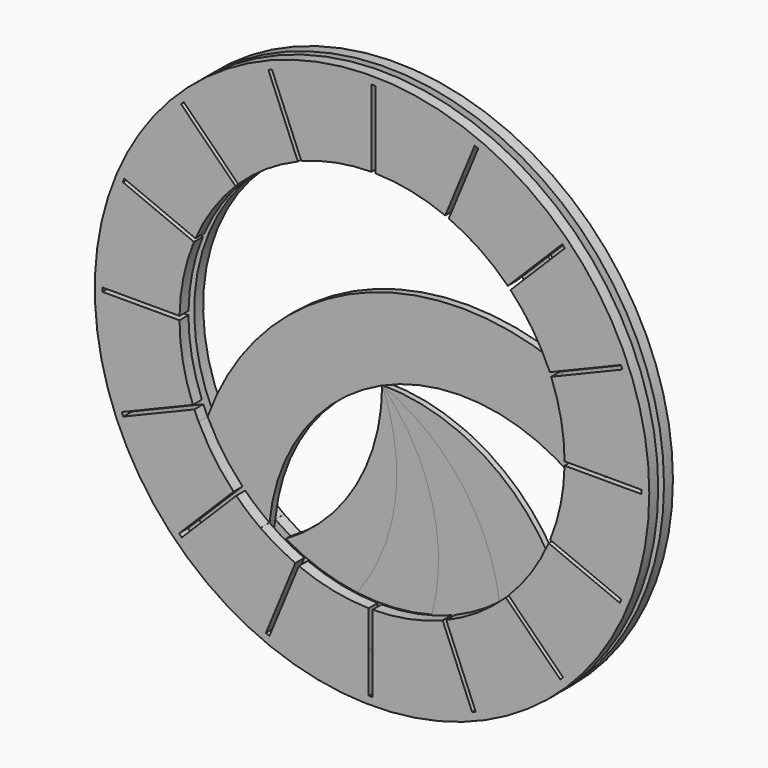
from build123d import *

# Parameters (mm, degrees)
F0_R      = 457.2
F0_R_2    = 444.5
F0_R_3    = 3.175
F1_DEPTH  = 18.415
F2_DEPTH  = 11.90625
F4_START  = 11.90625
F3_R      = 457.2
F3_R_2    = 3.175
F4_DEPTH  = 18.415
F5_R      = 3.175
F6_DEPTH  = 9.525
F7_DEPTH  = 9.525
F8_DEPTH  = 25.4
F9_DEPTH  = 9.525
F10_DEPTH = 9.525


with BuildPart() as f1:
    # F0 (on Front) → F1 (new body)
    with BuildSketch(Plane.XZ):
        Circle(F0_R)
        Circle(F0_R_2, mode=Mode.SUBTRACT)
        Circle(F0_R_2)
        with Locations((-145.8023877311, -351.9981018868)):
            Circle(F0_R_3, mode=Mode.SUBTRACT)
        with Locations((-351.9981018868, -145.8023877311)):
            Circle(F0_R_3, mode=Mode.SUBTRACT)
        with Locations((0, -381)):
            Circle(F0_R_3, mode=Mode.SUBTRACT)
        with Locations((145.8023877311, -351.9981018868)):
            Circle(F0_R_3, mode=Mode.SUBTRACT)
        with Locations((269.4076836321, -269.4076836321)):
            Circle(F0_R_3, mode=Mode.SUBTRACT)
        with BuildLine():
            ThreePointArc((422.4513888889, 48.1043902277), (438.7252682733, 26.4583333333), (444.5, 0))
            ThreePointArc((444.5, 0), (407.4583333333, -57.7252682733), (339.5486111111, -48.1043902277))
            ThreePointArc((339.5486111111, -48.1043902277), (328.041448396, -38.6497965609), (316.103577158, -29.7452266409))
            ThreePointArc((316.103577158, -29.7452266409), (132.2916666667, -288.6263413664), (-183.8119104913, -258.8811147255))
            ThreePointArc((-183.8119104913, -258.8811147255), (-183.9228426359, -260.0845455834), (-184.0291932426, -261.2883899749))
            ThreePointArc((-184.0291932426, -261.2883899749), (-252.7609555027, -319.0849716785), (-310.5575372063, -250.3532094184))
            ThreePointArc((-310.5575372063, -250.3532094184), (-301.8872628806, -193.3955315556), (-285.9227769911, -138.0377325143))
            ThreePointArc((-285.9227769911, -138.0377325143), (-132.2916666667, 288.6263413664), (291.2144436578, 126.4926788597))
            ThreePointArc((291.2144436578, 126.4926788596), (360.2279597917, 92.9824848895), (422.4513888889, 48.1043902277))
        make_face(mode=Mode.SUBTRACT)
        with Locations((351.9981018868, -145.8023877311)):
            Circle(F0_R_3, mode=Mode.SUBTRACT)
        with Locations((-381, 0)):
            Circle(F0_R_3, mode=Mode.SUBTRACT)
        with Locations((-351.9981018868, 145.8023877311)):
            Circle(F0_R_3, mode=Mode.SUBTRACT)
        with Locations((-269.4076836321, 269.4076836321)):
            Circle(F0_R_3, mode=Mode.SUBTRACT)
        with Locations((-145.8023877311, 351.9981018868)):
            Circle(F0_R_3, mode=Mode.SUBTRACT)
        with Locations((351.9981018868, 145.8023877311)):
            Circle(F0_R_3, mode=Mode.SUBTRACT)
        with Locations((0, 381)):
            Circle(F0_R_3, mode=Mode.SUBTRACT)
        with Locations((145.8023877311, 351.9981018868)):
            Circle(F0_R_3, mode=Mode.SUBTRACT)
        with Locations((269.4076836321, 269.4076836321)):
            Circle(F0_R_3, mode=Mode.SUBTRACT)
        with BuildLine():
            ThreePointArc((339.5486111111, -48.1043902277), (407.4583333333, -57.7252682733), (444.5, 0))
            ThreePointArc((444.5, 0), (438.7252682733, 26.4583333333), (422.4513888889, 48.1043902277))
            ThreePointArc((422.4513888889, 48.1043902277), (360.2279597917, 92.9824848895), (291.2144436578, 126.4926788596))
            ThreePointArc((291.2144436578, 126.4926788597), (310.8591609245, 64.597461787), (317.5, 0))
            ThreePointArc((317.5, 0), (317.1507021494, -14.8889934572), (316.103577158, -29.7452266409))
            ThreePointArc((316.103577158, -29.7452266409), (328.041448396, -38.6497965609), (339.5486111111, -48.1043902277))
        make_face()
        with Locations((381, 0)):
            Circle(F0_R_3, mode=Mode.SUBTRACT)
        with BuildLine():
            ThreePointArc((-183.8653331924, -258.8431750115), (-242.5359887763, -204.8964229759), (-285.9227769911, -138.0377325143))
            ThreePointArc((-285.9227769911, -138.0377325143), (-301.8872628806, -193.3955315556), (-310.5575372063, -250.3532094184))
            ThreePointArc((-310.5575372063, -250.3532094184), (-252.7609555027, -319.0849716785), (-184.0291932426, -261.2883899749))
            ThreePointArc((-184.0291932426, -261.2883899749), (-183.9354658864, -260.0665730623), (-183.8653331924, -258.8431750115))
        make_face()
        with Locations((-269.4076836321, -269.4076836321)):
            Circle(F0_R_3, mode=Mode.SUBTRACT)
        with Locations((-247.2933652244, -255.8207996967)):
            Circle(F0_R_3, mode=Mode.SUBTRACT)
        with Locations((-247.2933652244, -255.8207996967)):
            Circle(F0_R_3)
    extrude(amount=-F1_DEPTH)


with BuildPart() as f2:
    # F0 (on Front) → F2 (new body)
    with BuildSketch(Plane.XZ):
        with BuildLine():
            ThreePointArc((-183.8119104913, -258.8811147255), (0, 0), (316.103577158, -29.7452266409))
            ThreePointArc((316.103577158, -29.7452266409), (317.1507021494, -14.8889934572), (317.5, 0))
            ThreePointArc((317.5, 0), (310.8591609245, 64.597461787), (291.2144436578, 126.4926788597))
            ThreePointArc((291.2144436578, 126.4926788596), (-52.9166666667, 115.4505365466), (-285.9227769911, -138.0377325143))
            ThreePointArc((-285.9227769911, -138.0377325143), (-242.5359887763, -204.8964229759), (-183.8653331924, -258.8431750115))
            ThreePointArc((-183.8653331924, -258.8431750115), (-183.8386228206, -258.8621462467), (-183.8119104913, -258.8811147255))
        make_face()
        with BuildLine():
            ThreePointArc((339.5486111111, -48.1043902277), (407.4583333333, -57.7252682733), (444.5, 0))
            ThreePointArc((444.5, 0), (438.7252682733, 26.4583333333), (422.4513888889, 48.1043902277))
            ThreePointArc((422.4513888889, 48.1043902277), (360.2279597917, 92.9824848895), (291.2144436578, 126.4926788596))
            ThreePointArc((291.2144436578, 126.4926788597), (310.8591609245, 64.597461787), (317.5, 0))
            ThreePointArc((317.5, 0), (317.1507021494, -14.8889934572), (316.103577158, -29.7452266409))
            ThreePointArc((316.103577158, -29.7452266409), (328.041448396, -38.6497965609), (339.5486111111, -48.1043902277))
        make_face()
        with Locations((381, 0)):
            Circle(F0_R_3, mode=Mode.SUBTRACT)
        with BuildLine():
            ThreePointArc((-183.8653331924, -258.8431750115), (-242.5359887763, -204.8964229759), (-285.9227769911, -138.0377325143))
            ThreePointArc((-285.9227769911, -138.0377325143), (-301.8872628806, -193.3955315556), (-310.5575372063, -250.3532094184))
            ThreePointArc((-310.5575372063, -250.3532094184), (-252.7609555027, -319.0849716785), (-184.0291932426, -261.2883899749))
            ThreePointArc((-184.0291932426, -261.2883899749), (-183.9354658864, -260.0665730623), (-183.8653331924, -258.8431750115))
        make_face()
        with Locations((-269.4076836321, -269.4076836321)):
            Circle(F0_R_3, mode=Mode.SUBTRACT)
        with Locations((-247.2933652244, -255.8207996967)):
            Circle(F0_R_3, mode=Mode.SUBTRACT)
        with Locations((-269.4076836321, -269.4076836321)):
            Circle(F0_R_3)
    extrude(amount=F2_DEPTH)


with BuildPart() as f4:
    # F3 (on Front) → F4 (new body)
    with BuildSketch(Plane.XZ.offset(F4_START)):
        Circle(F3_R)
        with BuildLine():
            ThreePointArc((444.4991019176, 0.893529228), (444.4997754793, 0.4467648397), (444.5, 0))
            ThreePointArc((444.5, 0), (444.4916269754, -2.7282867786), (444.4665082171, -5.456470772))
            ThreePointArc((444.4665082171, -5.456470772), (435.5082100725, -88.9541958505), (411.0055613132, -169.2769286396))
            ThreePointArc((411.0055613132, -169.2769286396), (409.7859392208, -172.208402864), (408.5454088649, -175.1310906019))
            ThreePointArc((408.5454088649, -175.1310906019), (368.3158245353, -248.844737531), (314.9401497735, -313.6765086209))
            ThreePointArc((314.9401497735, -313.6765086209), (312.6915392669, -315.9181084884), (310.4269744864, -318.1435894549))
            ThreePointArc((310.4269744864, -318.1435894549), (245.0506935038, -370.8509237056), (170.9279553705, -410.3216836494))
            ThreePointArc((170.9279553705, -410.3216836494), (167.9926870155, -411.5321459003), (165.0488472698, -412.7216107922))
            ThreePointArc((165.0488472698, -412.7216107922), (84.4788157765, -436.398418518), (0.893529228, -444.4991019176))
            ThreePointArc((0.893529228, -444.4991019176), (-2.2815289766, -444.4941446471), (-5.456470772, -444.4665082171))
            ThreePointArc((-5.456470772, -444.4665082171), (-88.9541958505, -435.5082100725), (-169.2769286396, -411.0055613132))
            ThreePointArc((-169.2769286396, -411.0055613132), (-172.208402864, -409.7859392208), (-175.1310906019, -408.5454088649))
            ThreePointArc((-175.1310906019, -408.5454088649), (-248.844737531, -368.3158245353), (-313.6765086209, -314.9401497735))
            ThreePointArc((-313.6765086209, -314.9401497735), (-315.9181084884, -312.6915392669), (-318.1435894549, -310.4269744864))
            ThreePointArc((-318.1435894549, -310.4269744864), (-370.8509237056, -245.0506935038), (-410.3216836494, -170.9279553705))
            ThreePointArc((-410.3216836494, -170.9279553705), (-411.5321459003, -167.9926870155), (-412.7216107922, -165.0488472698))
            ThreePointArc((-412.7216107922, -165.0488472698), (-436.398418518, -84.4788157765), (-444.4991019176, -0.893529228))
            ThreePointArc((-444.4991019176, -0.893529228), (-444.4941446471, 2.2815289766), (-444.4665082171, 5.456470772))
            ThreePointArc((-444.4665082171, 5.456470772), (-435.5082100725, 88.9541958505), (-411.0055613132, 169.2769286396))
            ThreePointArc((-411.0055613132, 169.2769286396), (-409.7859392208, 172.208402864), (-408.5454088649, 175.1310906019))
            ThreePointArc((-408.5454088649, 175.1310906019), (-368.3158245353, 248.844737531), (-314.9401497735, 313.6765086209))
            ThreePointArc((-314.9401497735, 313.6765086209), (-312.6915392669, 315.9181084884), (-310.4269744864, 318.1435894549))
            ThreePointArc((-310.4269744864, 318.1435894549), (-245.0506935038, 370.8509237056), (-170.9279553705, 410.3216836494))
            ThreePointArc((-170.9279553705, 410.3216836494), (-167.9926870155, 411.5321459003), (-165.0488472698, 412.7216107922))
            ThreePointArc((-165.0488472698, 412.7216107922), (-84.4788157765, 436.398418518), (-0.893529228, 444.4991019176))
            ThreePointArc((-0.893529228, 444.4991019176), (2.2815289766, 444.4941446471), (5.456470772, 444.4665082171))
            ThreePointArc((5.456470772, 444.4665082171), (88.9541958505, 435.5082100725), (169.2769286396, 411.0055613132))
            ThreePointArc((169.2769286396, 411.0055613132), (172.208402864, 409.7859392208), (175.1310906019, 408.5454088649))
            ThreePointArc((175.1310906019, 408.5454088649), (248.844737531, 368.3158245353), (313.6765086209, 314.9401497735))
            ThreePointArc((313.6765086209, 314.9401497735), (315.9181084884, 312.6915392669), (318.1435894549, 310.4269744864))
            ThreePointArc((318.1435894549, 310.4269744864), (370.8509237056, 245.0506935038), (410.3216836494, 170.9279553705))
            ThreePointArc((410.3216836494, 170.9279553705), (411.5321459003, 167.9926870155), (412.7216107922, 165.0488472698))
            ThreePointArc((412.7216107922, 165.0488472698), (436.398418518, 84.4788157765), (444.4991019176, 0.893529228))
        make_face(mode=Mode.SUBTRACT)
        with BuildLine():
            ThreePointArc((0.893529228, -444.4991019176), (84.4788157765, -436.398418518), (165.0488472698, -412.7216107922))
            Line((165.0488472698, -412.7216107922), (116.4429240103, -295.3765316472))
            ThreePointArc((116.4429240103, -295.3765316472), (59.7018330532, -311.8364012268), (0.893529228, -317.4987426834))
            Line((0.893529228, -317.4987426834), (0.893529228, -444.4991019176))
        make_face()
        with BuildLine():
            ThreePointArc((-5.456470772, -317.4531098079), (-64.1773227466, -310.9461709767), (-120.6759952562, -293.6725287951))
            Line((-120.6759952562, -293.6725287951), (-169.2769286396, -411.0055613132))
            ThreePointArc((-169.2769286396, -411.0055613132), (-88.9541958505, -435.5082100725), (-5.456470772, -444.4665082171))
            Line((-5.456470772, -444.4665082171), (-5.456470772, -379.1493962176))
            ThreePointArc((-5.456470772, -379.1493962176), (-5.4858422756, -378.718529228), (-5.456470772, -378.2876622384))
            Line((-5.456470772, -378.2876622384), (-5.456470772, -317.4531098079))
        make_face()
        with BuildLine():
            ThreePointArc((170.9279553705, -410.3216836494), (245.0506935038, -370.8509237056), (310.4269744864, -318.1435894549))
            Line((310.4269744864, -318.1435894549), (220.6149391697, -228.3315541382))
            ThreePointArc((220.6149391697, -228.3315541382), (174.4919259691, -265.2523661941), (122.3270219871, -292.9886511313))
            Line((122.3270219871, -292.9886511313), (144.9919439166, -347.7066130437))
            ThreePointArc((144.9919439166, -347.7066130437), (146.3432423245, -348.8781658945), (146.8469499574, -350.5942142883))
            ThreePointArc((146.8469499574, -350.5942142883), (146.7966055901, -351.1573769442), (146.6471690585, -351.70268003))
            Line((146.6471690585, -351.70268003), (170.9279553705, -410.3216836494))
        make_face()
        with BuildLine():
            Line((146.6307933887, 356.3329544552), (169.2769286396, 411.0055613132))
            ThreePointArc((169.2769286396, 411.0055613132), (88.9541958505, 435.5082100725), (5.456470772, 444.4665082171))
            Line((5.456470772, 444.4665082171), (5.456470772, 383.3108422756))
            Line((5.456470772, 383.3108422756), (5.456470772, 317.4531098079))
            ThreePointArc((5.456470772, 317.4531098079), (64.1773227466, 310.9461709767), (120.6759952562, 293.6725287951))
            Line((120.6759952562, 293.6725287951), (144.9535218219, 352.2836626909))
            ThreePointArc((144.9535218219, 352.2836626909), (144.9813764733, 354.6441451141), (146.6307933887, 356.3329544552))
        make_face()
        with BuildLine():
            Line((-0.893529228, 383.3108422756), (-0.893529228, 444.4991019176))
            ThreePointArc((-0.893529228, 444.4991019176), (-84.4788157765, 436.398418518), (-165.0488472698, 412.7216107922))
            Line((-165.0488472698, 412.7216107922), (-142.4203824907, 358.0916642267))
            ThreePointArc((-142.4203824907, 358.0916642267), (-141.0416592427, 356.9205463337), (-140.526321461, 355.1865273359))
            ThreePointArc((-140.526321461, 355.1865273359), (-140.5805336323, 354.6023113415), (-140.7413188331, 354.0380459723))
            Line((-140.7413188331, 354.0380459723), (-116.4429240103, 295.3765316472))
            ThreePointArc((-116.4429240103, 295.3765316472), (-59.7018330532, 311.8364012268), (-0.893529228, 317.4987426834))
            Line((-0.893529228, 317.4987426834), (-0.893529228, 383.3108422756))
        make_face()
        with BuildLine():
            ThreePointArc((314.9401497735, -313.6765086209), (368.3158245353, -248.844737531), (408.5454088649, -175.1310906019))
            Line((408.5454088649, -175.1310906019), (291.20032972, -126.5251673423))
            ThreePointArc((291.20032972, -126.5251673423), (262.7172049295, -178.2860629271), (225.1373345459, -223.8736933933))
            Line((225.1373345459, -223.8736933933), (266.9456916083, -265.6820504557))
            ThreePointArc((266.9456916083, -265.6820504557), (269.7075090207, -266.2227656353), (270.9547544263, -268.7455393516))
            ThreePointArc((270.9547544263, -268.7455393516), (270.9267531747, -269.1662814076), (270.8432433222, -269.5796021696))
            Line((270.8432433222, -269.5796021696), (314.9401497735, -313.6765086209))
        make_face()
        with BuildLine():
            Line((271.8840859169, 273.1477270695), (313.6765086209, 314.9401497735))
            ThreePointArc((313.6765086209, 314.9401497735), (248.844737531, 368.3158245353), (175.1310906019, 408.5454088649))
            Line((175.1310906019, 408.5454088649), (126.5251673423, 291.20032972))
            ThreePointArc((126.5251673423, 291.20032972), (178.2860629271, 262.7172049295), (223.8736933933, 225.1373345459))
            Line((223.8736933933, 225.1373345459), (267.969879756, 269.2335209086))
            ThreePointArc((267.969879756, 269.2335209086), (268.7819460933, 272.3356607322), (271.8840859169, 273.1477270695))
        make_face()
        with BuildLine():
            Line((-122.3270219871, 292.9886511313), (-170.9279553705, 410.3216836494))
            ThreePointArc((-170.9279553705, 410.3216836494), (-245.0506935038, 370.8509237056), (-310.4269744864, 318.1435894549))
            Line((-310.4269744864, 318.1435894549), (-268.6756914301, 276.3923063985))
            ThreePointArc((-268.6756914301, 276.3923063985), (-265.8948010441, 275.8708319158), (-264.6341259299, 273.3378523992))
            ThreePointArc((-264.6341259299, 273.3378523992), (-264.664406829, 272.9003975146), (-264.7546719306, 272.4712868991))
            Line((-264.7546719306, 272.4712868991), (-220.6149391697, 228.3315541382))
            ThreePointArc((-220.6149391697, 228.3315541382), (-174.4919259691, 265.2523661941), (-122.3270219871, 292.9886511313))
        make_face()
        with BuildLine():
            Line((-347.9778941764, 150.0432045786), (-291.20032972, 126.5251673423))
            ThreePointArc((-291.20032972, 126.5251673423), (-262.7172049295, 178.2860629271), (-225.1373345459, 223.8736933933))
            Line((-225.1373345459, 223.8736933933), (-314.9401497735, 313.6765086209))
            ThreePointArc((-314.9401497735, 313.6765086209), (-368.3158245353, 248.844737531), (-408.5454088649, 175.1310906019))
            Line((-408.5454088649, 175.1310906019), (-353.5179413961, 152.3379672732))
            ThreePointArc((-353.5179413961, 152.3379672732), (-350.0173969675, 153.1925453708), (-347.9726544443, 150.2255362646))
            ThreePointArc((-347.9726544443, 150.2255362646), (-347.9739646477, 150.1343327854), (-347.9778941764, 150.0432045786))
        make_face()
        with BuildLine():
            Line((-350.5268722304, -139.2869430493), (-295.3765316472, -116.4429240103))
            ThreePointArc((-295.3765316472, -116.4429240103), (-311.8364012268, -59.7018330532), (-317.4987426834, -0.893529228))
            Line((-317.4987426834, -0.893529228), (-444.4991019176, -0.893529228))
            ThreePointArc((-444.4991019176, -0.893529228), (-436.398418518, -84.4788157765), (-412.7216107922, -165.0488472698))
            Line((-412.7216107922, -165.0488472698), (-356.0741114993, -141.5846847882))
            ThreePointArc((-356.0741114993, -141.5846847882), (-354.1200764617, -138.4571616697), (-350.5268722304, -139.2869430493))
        make_face()
        with BuildLine():
            Line((-377.9742354301, 5.456470772), (-317.4531098079, 5.456470772))
            ThreePointArc((-317.4531098079, 5.456470772), (-310.9461709767, 64.1773227466), (-293.6725287951, 120.6759952562))
            Line((-293.6725287951, 120.6759952562), (-411.0055613132, 169.2769286396))
            ThreePointArc((-411.0055613132, 169.2769286396), (-435.5082100725, 88.9541958505), (-444.4665082171, 5.456470772))
            Line((-444.4665082171, 5.456470772), (-384.0845075771, 5.456470772))
            ThreePointArc((-384.0845075771, 5.456470772), (-381.0293715036, 7.7673130476), (-377.9742354301, 5.456470772))
        make_face()
        with BuildLine():
            Line((355.2331404575, 148.109533649), (410.3216836494, 170.9279553705))
            ThreePointArc((410.3216836494, 170.9279553705), (370.8509237056, 245.0506935038), (318.1435894549, 310.4269744864))
            Line((318.1435894549, 310.4269744864), (228.3315541382, 220.6149391697))
            ThreePointArc((228.3315541382, 220.6149391697), (264.0014411474, 176.3788226293), (291.2144436578, 126.4926788596))
            ThreePointArc((291.2144436578, 126.4926788596), (294.2607523904, 125.3135881763), (297.2983140397, 124.112142813))
            Line((297.2983140397, 124.112142813), (349.7048790855, 145.8196528124))
            ThreePointArc((349.7048790855, 145.8196528124), (351.6606651625, 148.9161097488), (355.2331404575, 148.109533649))
        make_face()
        with BuildLine():
            ThreePointArc((411.0055613132, -169.2769286396), (435.5082100725, -88.9541958505), (444.4665082171, -5.456470772))
            Line((444.4665082171, -5.456470772), (444.2651319979, -5.456470772))
            ThreePointArc((444.2651319979, -5.456470772), (404.951432224, -58.8096836789), (339.5486111111, -48.1043902277))
            ThreePointArc((339.5486111111, -48.1043902277), (328.041448396, -38.6497965609), (316.103577158, -29.7452266409))
            ThreePointArc((316.103577158, -29.7452266409), (308.2593486305, -76.0422512944), (293.6725287951, -120.6759952562))
            Line((293.6725287951, -120.6759952562), (348.7688393659, -143.4976343313))
            ThreePointArc((348.7688393659, -143.4976343313), (352.2630845938, -142.6717954912), (354.2932829407, -145.633223217))
            ThreePointArc((354.2932829407, -145.633223217), (354.2923820296, -145.7088537277), (354.2896798074, -145.7844413179))
            Line((354.2896798074, -145.7844413179), (411.0055613132, -169.2769286396))
        make_face()
        with BuildLine():
            ThreePointArc((-126.5251673423, -291.20032972), (-156.0077189886, -276.5281931666), (-183.8119104913, -258.8811147255))
            ThreePointArc((-183.8119104913, -258.8811147255), (-183.9228426359, -260.0845455834), (-184.0291932426, -261.2883899749))
            ThreePointArc((-184.0291932426, -261.2883899749), (-227.9761851143, -316.3112663224), (-295.6794161791, -296.9430573317))
            Line((-295.6794161791, -296.9430573317), (-313.6765086209, -314.9401497735))
            ThreePointArc((-313.6765086209, -314.9401497735), (-248.844737531, -368.3158245353), (-175.1310906019, -408.5454088649))
            Line((-175.1310906019, -408.5454088649), (-150.889729434, -350.0215859632))
            ThreePointArc((-150.889729434, -350.0215859632), (-150.8773830083, -347.621792271), (-149.1892028564, -345.9161516364))
            Line((-149.1892028564, -345.9161516364), (-126.5251673423, -291.20032972))
        make_face()
        with BuildLine():
            ThreePointArc((-310.5575372063, -250.3532094184), (-301.8872628806, -193.3955315555), (-285.9227769911, -138.0377325143))
            ThreePointArc((-285.9227769911, -138.0377325143), (-289.5622851979, -130.2303074978), (-292.9886511313, -122.3270219871))
            Line((-292.9886511313, -122.3270219871), (-410.3216836494, -170.9279553705))
            ThreePointArc((-410.3216836494, -170.9279553705), (-370.8509237056, -245.0506935038), (-318.1435894549, -310.4269744864))
            Line((-318.1435894549, -310.4269744864), (-299.5759800047, -291.8593650362))
            ThreePointArc((-299.5759800047, -291.8593650362), (-308.6811101032, -272.062560029), (-310.5575372063, -250.3532094184))
        make_face()
        with BuildLine():
            Line((384.0466753222, 0.893529228), (444.4937131181, 0.893529228))
            ThreePointArc((444.4937131181, 0.893529228), (438.5376829382, 26.863824041), (422.4513888889, 48.1043902277))
            ThreePointArc((422.4513888889, 48.1043902277), (366.8608063144, 88.9416243363), (305.6214900159, 120.6865247125))
            Line((305.6214900159, 120.6865247125), (295.3765316472, 116.4429240103))
            ThreePointArc((295.3765316472, 116.4429240103), (311.8364012268, 59.7018330532), (317.4987426834, 0.893529228))
            Line((317.4987426834, 0.893529228), (377.9533246778, 0.893529228))
            ThreePointArc((377.9533246778, 0.893529228), (381, 3.175), (384.0466753222, 0.893529228))
        make_face()
        with BuildLine():
            Line((444.4937131181, 0.893529228), (444.4991019176, 0.893529228))
            ThreePointArc((444.4991019176, 0.893529228), (436.398418518, 84.4788157765), (412.7216107922, 165.0488472698))
            Line((412.7216107922, 165.0488472698), (305.6214900159, 120.6865247125))
            ThreePointArc((305.6214900159, 120.6865247125), (366.8608063144, 88.9416243363), (422.4513888889, 48.1043902277))
            ThreePointArc((422.4513888889, 48.1043902277), (438.5376829382, 26.863824041), (444.4937131181, 0.893529228))
        make_face()
        with BuildLine():
            ThreePointArc((-228.3315541382, -220.6149391697), (-260.4210591255, -181.6235721594), (-285.9227769911, -138.0377325143))
            ThreePointArc((-285.9227769911, -138.0377325143), (-301.8872628806, -193.3955315555), (-310.5575372063, -250.3532094184))
            ThreePointArc((-310.5575372063, -250.3532094184), (-308.6811101032, -272.062560029), (-299.5759800047, -291.8593650362))
            Line((-299.5759800047, -291.8593650362), (-274.1042725424, -266.387657574))
            ThreePointArc((-274.1042725424, -266.387657574), (-273.3014456575, -263.253219624), (-270.1670077076, -262.4503927391))
            Line((-270.1670077076, -262.4503927391), (-228.3315541382, -220.6149391697))
        make_face()
        with BuildLine():
            ThreePointArc((-184.0291932426, -261.2883899749), (-183.9354658864, -260.0665730623), (-183.8653331924, -258.8431750115))
            ThreePointArc((-183.8653331924, -258.8431750115), (-204.5649025875, -242.8156721247), (-223.8736933933, -225.1373345459))
            Line((-223.8736933933, -225.1373345459), (-295.6794161791, -296.9430573317))
            ThreePointArc((-295.6794161791, -296.9430573317), (-227.9761851143, -316.3112663224), (-184.0291932426, -261.2883899749))
        make_face()
        with Locations((-247.2933652244, -255.8207996967)):
            Circle(F3_R_2, mode=Mode.SUBTRACT)
        with BuildLine():
            ThreePointArc((339.5486111111, -48.1043902277), (404.951432224, -58.8096836789), (444.2651319979, -5.456470772))
            Line((444.2651319979, -5.456470772), (317.4531098079, -5.456470772))
            ThreePointArc((317.4531098079, -5.456470772), (317.0110484119, -17.6137782653), (316.103577158, -29.7452266409))
            ThreePointArc((316.103577158, -29.7452266409), (328.041448396, -38.6497965609), (339.5486111111, -48.1043902277))
        make_face()
        with Locations((-247.2933652244, -255.8207996967)):
            Circle(F3_R_2)
        with BuildLine():
            Line((292.9886511313, 122.3270219871), (297.2983140397, 124.112142813))
            ThreePointArc((297.2983140397, 124.112142813), (294.2607523904, 125.3135881763), (291.2144436578, 126.4926788596))
            ThreePointArc((291.2144436578, 126.4926788596), (292.1089730984, 124.4130131273), (292.9886511313, 122.3270219871))
        make_face()
        with BuildLine():
            Line((-384.0845075771, 5.456470772), (-377.9742354301, 5.456470772))
            ThreePointArc((-377.9742354301, 5.456470772), (-381.0293715036, 7.7673130476), (-384.0845075771, 5.456470772))
        make_face()
        with BuildLine():
            Line((377.9533246778, 0.893529228), (384.0466753222, 0.893529228))
            ThreePointArc((384.0466753222, 0.893529228), (381, 3.175), (377.9533246778, 0.893529228))
        make_face()
        with BuildLine():
            Line((-356.0741114993, -141.5846847882), (-350.5268722304, -139.2869430493))
            ThreePointArc((-350.5268722304, -139.2869430493), (-354.1200764617, -138.4571616697), (-356.0741114993, -141.5846847882))
        make_face()
        with BuildLine():
            Line((-353.5179413961, 152.3379672732), (-347.9778941764, 150.0432045786))
            ThreePointArc((-347.9778941764, 150.0432045786), (-347.9739646477, 150.1343327854), (-347.9726544443, 150.2255362646))
            ThreePointArc((-347.9726544443, 150.2255362646), (-350.0173969675, 153.1925453708), (-353.5179413961, 152.3379672732))
        make_face()
        with BuildLine():
            Line((349.7048790855, 145.8196528124), (355.2331404575, 148.109533649))
            ThreePointArc((355.2331404575, 148.109533649), (351.6606651625, 148.9161097488), (349.7048790855, 145.8196528124))
        make_face()
        with BuildLine():
            Line((348.7688393659, -143.4976343313), (354.2896798074, -145.7844413179))
            ThreePointArc((354.2896798074, -145.7844413179), (354.2923820296, -145.7088537277), (354.2932829407, -145.633223217))
            ThreePointArc((354.2932829407, -145.633223217), (352.2630845938, -142.6717954912), (348.7688393659, -143.4976343313))
        make_face()
        with BuildLine():
            Line((-274.1042725424, -266.387657574), (-270.1670077076, -262.4503927391))
            ThreePointArc((-270.1670077076, -262.4503927391), (-273.3014456575, -263.253219624), (-274.1042725424, -266.387657574))
        make_face()
        with BuildLine():
            ThreePointArc((-264.6341259299, 273.3378523992), (-265.8948010441, 275.8708319158), (-268.6756914301, 276.3923063985))
            Line((-268.6756914301, 276.3923063985), (-264.7546719306, 272.4712868991))
            ThreePointArc((-264.7546719306, 272.4712868991), (-264.664406829, 272.9003975146), (-264.6341259299, 273.3378523992))
        make_face()
        with BuildLine():
            Line((267.969879756, 269.2335209086), (271.8840859169, 273.1477270695))
            ThreePointArc((271.8840859169, 273.1477270695), (268.7819460933, 272.3356607322), (267.969879756, 269.2335209086))
        make_face()
        with BuildLine():
            Line((266.9456916083, -265.6820504557), (270.8432433222, -269.5796021696))
            ThreePointArc((270.8432433222, -269.5796021696), (270.9267531747, -269.1662814076), (270.9547544263, -268.7455393516))
            ThreePointArc((270.9547544263, -268.7455393516), (269.7075090207, -266.2227656353), (266.9456916083, -265.6820504557))
        make_face()
        with BuildLine():
            Line((-150.889729434, -350.0215859632), (-149.1892028564, -345.9161516364))
            ThreePointArc((-149.1892028564, -345.9161516364), (-150.8773830083, -347.621792271), (-150.889729434, -350.0215859632))
        make_face()
        with BuildLine():
            ThreePointArc((-140.526321461, 355.1865273359), (-141.0416592427, 356.9205463337), (-142.4203824907, 358.0916642267))
            Line((-142.4203824907, 358.0916642267), (-140.7413188331, 354.0380459723))
            ThreePointArc((-140.7413188331, 354.0380459723), (-140.5805336323, 354.6023113415), (-140.526321461, 355.1865273359))
        make_face()
        with BuildLine():
            Line((144.9535218219, 352.2836626909), (146.6307933887, 356.3329544552))
            ThreePointArc((146.6307933887, 356.3329544552), (144.9813764733, 354.6441451141), (144.9535218219, 352.2836626909))
        make_face()
        with BuildLine():
            Line((144.9919439166, -347.7066130437), (146.6471690585, -351.70268003))
            ThreePointArc((146.6471690585, -351.70268003), (146.7966055901, -351.1573769442), (146.8469499574, -350.5942142883))
            ThreePointArc((146.8469499574, -350.5942142883), (146.3432423245, -348.8781658945), (144.9919439166, -347.7066130437))
        make_face()
    extrude(amount=F4_DEPTH)


with BuildPart() as f6:
    # F5 (on Front) → F6 (new body)
    with BuildSketch(Plane.XZ):
        with BuildLine():
            ThreePointArc((71.7370250666, -375.0863708473), (104.2081806235, -413.9328112946), (154.7634294478, -416.6875698957))
            ThreePointArc((154.7634294478, -416.6875698957), (166.2544105163, -411.0429346054), (176.3796033569, -403.2080751032))
            ThreePointArc((176.3796033569, -403.2080751032), (186.4354217322, -370.6673875603), (192.9476872854, -337.2367694635))
            ThreePointArc((192.9476872854, -337.2367694635), (162.4728125061, -301.0973226443), (115.4717831233, -296.0296953712))
            ThreePointArc((115.4717831233, -296.0296953712), (95.6182169929, -336.6720898203), (71.7370250666, -375.0863708473))
        make_face()
        with Locations((132.6543703377, -357.1607733645)):
            Circle(F5_R, mode=Mode.SUBTRACT)
        with Locations((145.8023877311, -351.9981018868)):
            Circle(F5_R, mode=Mode.SUBTRACT)
        with Locations((145.8023877311, -351.9981018868)):
            Circle(F5_R)
        with BuildLine():
            ThreePointArc((73.1275733638, -335.0517154464), (69.1926396762, -354.9565180605), (71.7370250666, -375.0863708473))
            ThreePointArc((71.7370250666, -375.0863708473), (95.6182169929, -336.6720898203), (115.4717831233, -296.0296953712))
            ThreePointArc((115.4717831233, -296.0296953712), (112.9921770152, -296.7815703741), (110.5453087818, -297.6339777417))
            ThreePointArc((110.5453087818, -297.6339777417), (87.7530883604, -312.2594941311), (73.1275733638, -335.0517154464))
        make_face()
        with BuildLine():
            ThreePointArc((176.3796033569, -403.2080751032), (185.6497015444, -392.1428383448), (192.1811652363, -379.2698368702))
            ThreePointArc((192.1811652363, -379.2698368702), (195.1531762306, -368.3923922135), (196.1543703377, -357.1607733645))
            ThreePointArc((196.1543703377, -357.1607733645), (195.3475742205, -347.0705708436), (192.9476872854, -337.2367694635))
            ThreePointArc((192.9476872854, -337.2367694635), (186.4354217322, -370.6673875603), (176.3796033569, -403.2080751032))
        make_face()
        with BuildLine():
            ThreePointArc((195.9980102241, -293.3317515723), (195.9434551289, -287.4462176822), (195.7798085915, -281.5627063802))
            ThreePointArc((195.7798085915, -281.5627063802), (194.8788477302, -266.6968936054), (193.2817537103, -251.8896855425))
            ThreePointArc((193.2817537103, -251.8896855425), (155.992293345, -276.5368952183), (115.611051916, -295.7031191497))
            ThreePointArc((115.611051916, -295.7031191497), (115.5414501251, -295.8664211651), (115.4717831233, -296.0296953712))
            ThreePointArc((115.4717831233, -296.0296953712), (162.4728125061, -301.0973226443), (192.9476872854, -337.2367694635))
            ThreePointArc((192.9476872854, -337.2367694635), (195.2345114889, -315.3371774149), (195.9980102241, -293.3317515723))
        make_face()
        with BuildLine():
            ThreePointArc((115.611051916, -295.7031191497), (155.992293345, -276.5368952183), (193.2817537103, -251.8896855425))
            ThreePointArc((193.2817537103, -251.8896855425), (178.3833346319, -189.0482811429), (151.0767247229, -130.5217567865))
            ThreePointArc((151.0767247229, -130.5217567865), (141.2638331902, -214.8129093132), (115.611051916, -295.7031191497))
        make_face()
        with BuildLine():
            ThreePointArc((110.5453087818, -297.6339777417), (113.082301554, -296.6793607167), (115.611051916, -295.7031191497))
            ThreePointArc((115.611051916, -295.7031191497), (141.2638331902, -214.8129093132), (151.0767247229, -130.5217567865))
            ThreePointArc((151.0767247229, -130.5217567865), (135.8509851339, -107.3863394078), (118.6669550389, -85.6658469406))
            ThreePointArc((118.6669550389, -85.6658469406), (106.6893686763, -132.8293247065), (89.628179925, -178.4009392099))
            ThreePointArc((89.628179925, -178.4009392099), (92.1511249804, -201.3923389873), (92.9935969733, -224.5064030267))
            ThreePointArc((92.9935969733, -224.5064030267), (90.2773404595, -265.9484690566), (82.17504682, -306.6814498468))
            ThreePointArc((82.17504682, -306.6814498468), (96.4663052765, -302.4904989356), (110.5453087818, -297.6339777417))
        make_face()
        with BuildLine():
            ThreePointArc((82.17504682, -306.6814498468), (77.9840953193, -320.9727101518), (73.1275733638, -335.0517154464))
            ThreePointArc((73.1275733638, -335.0517154464), (87.7530883604, -312.2594941311), (110.5453087818, -297.6339777417))
            ThreePointArc((110.5453087818, -297.6339777417), (96.4663052765, -302.4904989356), (82.17504682, -306.6814498468))
        make_face()
        with BuildLine():
            ThreePointArc((118.6669550389, -85.6658469406), (64.3369877421, -35.9019078575), (0, 0))
            ThreePointArc((0, 0), (59.2016365522, -81.9722026455), (89.628179925, -178.4009392099))
            ThreePointArc((89.628179925, -178.4009392099), (106.6893686763, -132.8293247065), (118.6669550389, -85.6658469406))
        make_face()
        with BuildLine():
            ThreePointArc((115.4717831233, -296.0296953712), (115.5414501251, -295.8664211651), (115.611051916, -295.7031191497))
            ThreePointArc((115.611051916, -295.7031191497), (113.082301554, -296.6793607167), (110.5453087818, -297.6339777417))
            ThreePointArc((110.5453087818, -297.6339777417), (112.9921770152, -296.7815703741), (115.4717831233, -296.0296953712))
        make_face()
    extrude(amount=F6_DEPTH)


with BuildPart() as f7:
    # F5 (on Front) → F7 (new body)
    with BuildSketch(Plane.XZ):
        with BuildLine():
            ThreePointArc((209.8157090115, -319.0820499696), (254.6810361529, -342.5453080894), (302.4421971995, -325.7437142189))
            ThreePointArc((302.4421971995, -325.7437142189), (310.8983692725, -316.1313442045), (317.2545556317, -305.0181359193))
            ThreePointArc((317.2545556317, -305.0181359193), (314.0921384109, -271.1062656334), (307.3153435864, -237.7282656803))
            ThreePointArc((307.3153435864, -237.7282656803), (265.3302629693, -216.0020001292), (219.9676769168, -229.3066382621))
            ThreePointArc((219.9676769168, -229.3066382621), (217.1785445289, -274.4529454773), (209.8157090115, -319.0820499696))
        make_face()
        with Locations((259.1133415959, -279.322888799)):
            Circle(F5_R, mode=Mode.SUBTRACT)
        with Locations((269.4076836321, -269.4076836321)):
            Circle(F5_R, mode=Mode.SUBTRACT)
        with BuildLine():
            ThreePointArc((195.7798085915, -281.5627063802), (199.7616413788, -301.4581827422), (209.8157090115, -319.0820499696))
            ThreePointArc((209.8157090115, -319.0820499696), (217.1785445289, -274.4529454773), (219.9676769168, -229.3066382621))
            ThreePointArc((219.9676769168, -229.3066382621), (217.9645498477, -230.9501842312), (216.0301406902, -232.6740817396))
            ThreePointArc((216.0301406902, -232.6740817396), (200.5698183044, -254.9084998687), (195.7798085915, -281.5627063802))
        make_face()
        with BuildLine():
            ThreePointArc((307.3153435864, -237.7282656803), (314.0921384109, -271.1062656334), (317.2545556317, -305.0181359193))
            ThreePointArc((317.2545556317, -305.0181359193), (321.3506496932, -292.4013662128), (322.7361683105, -279.2088985683))
            ThreePointArc((322.7361683105, -279.2088985683), (322.725257326, -278.0317936518), (322.692528122, -276.855093251))
            ThreePointArc((322.692528122, -276.855093251), (318.335838832, -255.9822125314), (307.3153435864, -237.7282656803))
        make_face()
        with Locations((269.4076836321, -269.4076836321)):
            Circle(F5_R)
        with BuildLine():
            ThreePointArc((193.2817537103, -251.8896855425), (194.8788477302, -266.6968936054), (195.7798085915, -281.5627063802))
            ThreePointArc((195.7798085915, -281.5627063802), (200.5698183044, -254.9084998687), (216.0301406902, -232.6740817396))
            ThreePointArc((216.0301406902, -232.6740817396), (204.8813475693, -242.5487238025), (193.2817537103, -251.8896855425))
        make_face()
        with BuildLine():
            ThreePointArc((216.0301406902, -232.6740817396), (218.0087001152, -230.8212656453), (219.9713691946, -228.9516253156))
            ThreePointArc((219.9713691946, -228.9516253156), (219.9880399939, -226.7290419578), (219.9935969733, -224.5064030267))
            ThreePointArc((219.9935969733, -224.5064030267), (212.3100921781, -142.2166739171), (189.5252076957, -62.771820075))
            ThreePointArc((189.5252076957, -62.771820075), (166.6049175904, -47.2241197689), (142.4168712896, -33.733044961))
            ThreePointArc((142.4168712896, -33.733044961), (148.9749931547, -77.3999085446), (151.1682484277, -121.5019897759))
            ThreePointArc((151.1682484277, -121.5019897759), (151.1453669125, -126.0121054483), (151.0767247229, -130.5217567865))
            ThreePointArc((151.0767247229, -130.5217567865), (178.3833346319, -189.0482811429), (193.2817537103, -251.8896855425))
            ThreePointArc((193.2817537103, -251.8896855425), (204.8813475693, -242.5487238025), (216.0301406902, -232.6740817396))
        make_face()
        with BuildLine():
            ThreePointArc((219.9713691946, -228.9516253156), (249.9441752887, -195.7911112366), (274.9630657016, -158.75))
            ThreePointArc((274.9630657016, -158.75), (237.150356918, -106.3934908306), (189.5252076957, -62.771820075))
            ThreePointArc((189.5252076957, -62.771820075), (212.3100921781, -142.2166739171), (219.9935969733, -224.5064030267))
            ThreePointArc((219.9935969733, -224.5064030267), (219.9880399939, -226.7290419578), (219.9713691946, -228.9516253156))
        make_face()
        with BuildLine():
            ThreePointArc((307.3153435864, -237.7282656803), (293.8050852065, -197.1470943151), (274.9630657016, -158.75))
            ThreePointArc((274.9630657016, -158.75), (249.9441752887, -195.7911112366), (219.9713691946, -228.9516253156))
            ThreePointArc((219.9713691946, -228.9516253156), (219.9695585003, -229.1291321575), (219.9676769168, -229.3066382621))
            ThreePointArc((219.9676769168, -229.3066382621), (265.3302629693, -216.0020001292), (307.3153435864, -237.7282656803))
        make_face()
        with BuildLine():
            ThreePointArc((151.1682484277, -121.5019897759), (148.9749931547, -77.3999085446), (142.4168712896, -33.733044961))
            ThreePointArc((142.4168712896, -33.733044961), (134.3760811411, -29.8381867241), (126.2288842292, -26.1711157708))
            ThreePointArc((126.2288842292, -26.1711157708), (123.4524665421, -56.0461617811), (118.6669550389, -85.6658469406))
            ThreePointArc((118.6669550389, -85.6658469406), (135.8509851339, -107.3863394078), (151.0767247229, -130.5217567865))
            ThreePointArc((151.0767247229, -130.5217567865), (151.1453669125, -126.0121054483), (151.1682484277, -121.5019897759))
        make_face()
        with BuildLine():
            ThreePointArc((118.6669550389, -85.6658469406), (123.4524665421, -56.0461617811), (126.2288842292, -26.1711157708))
            ThreePointArc((126.2288842292, -26.1711157708), (64.4566880053, -6.6116191116), (0, 0))
            ThreePointArc((0, 0), (64.3369877421, -35.9019078575), (118.6669550389, -85.6658469406))
        make_face()
        with BuildLine():
            ThreePointArc((219.9676769168, -229.3066382621), (219.9695585003, -229.1291321575), (219.9713691946, -228.9516253156))
            ThreePointArc((219.9713691946, -228.9516253156), (218.0087001152, -230.8212656453), (216.0301406902, -232.6740817396))
            ThreePointArc((216.0301406902, -232.6740817396), (217.9645498477, -230.9501842312), (219.9676769168, -229.3066382621))
        make_face()
    extrude(amount=F7_DEPTH)


with BuildPart() as f8:
    # F5 (on Front) → F8 (new body, symmetric)
    with BuildSketch(Plane.XZ):
        with Locations((381, 0)):
            Circle(F5_R)
    extrude(amount=F8_DEPTH, both=True)


with BuildPart() as f9:
    # F5 (on Front) → F9 (new body)
    with BuildSketch(Plane.XZ):
        with BuildLine():
            ThreePointArc((24.1682484277, -121.5019897759), (18.0675749557, -59.5608125358), (0, 0))
            ThreePointArc((0, 0), (-42.5369342984, -158.75), (-158.75, -274.9630657016))
            ThreePointArc((-158.75, -274.9630657016), (-102.0570302337, -300.6503161147), (-41.4420660299, -314.7837434862))
            ThreePointArc((-41.4420660299, -314.7837434862), (7.3185645424, -223.5590200097), (24.1682484277, -121.5019897759))
        make_face()
    extrude(amount=F9_DEPTH)


with BuildPart() as f10:
    # F5 (on Front) → F10 (new body)
    with BuildSketch(Plane.XZ):
        with BuildLine():
            ThreePointArc((92.9935969733, -224.5064030267), (92.1511249804, -201.3923389873), (89.628179925, -178.4009392099))
            ThreePointArc((89.628179925, -178.4009392099), (48.3054227162, -252.5205787879), (-6.35, -317.4364936487))
            ThreePointArc((-6.35, -317.4364936487), (38.2919988132, -315.1824437162), (82.17504682, -306.6814498468))
            ThreePointArc((82.17504682, -306.6814498468), (90.2773404595, -265.9484690566), (92.9935969733, -224.5064030267))
        make_face()
        with BuildLine():
            ThreePointArc((89.628179925, -178.4009392099), (59.2016365522, -81.9722026455), (0, 0))
            ThreePointArc((0, 0), (18.0675749557, -59.5608125358), (24.1682484277, -121.5019897759))
            ThreePointArc((24.1682484277, -121.5019897759), (7.3185645424, -223.5590200097), (-41.4420660299, -314.7837434862))
            ThreePointArc((-41.4420660299, -314.7837434862), (-23.9328156452, -316.5966998174), (-6.35, -317.4364936487))
            ThreePointArc((-6.35, -317.4364936487), (48.3054227162, -252.5205787879), (89.628179925, -178.4009392099))
        make_face()
    extrude(amount=F10_DEPTH)


solid = Compound([f1.part, f2.part, f4.part, f6.part, f7.part, f8.part, f9.part, f10.part])
